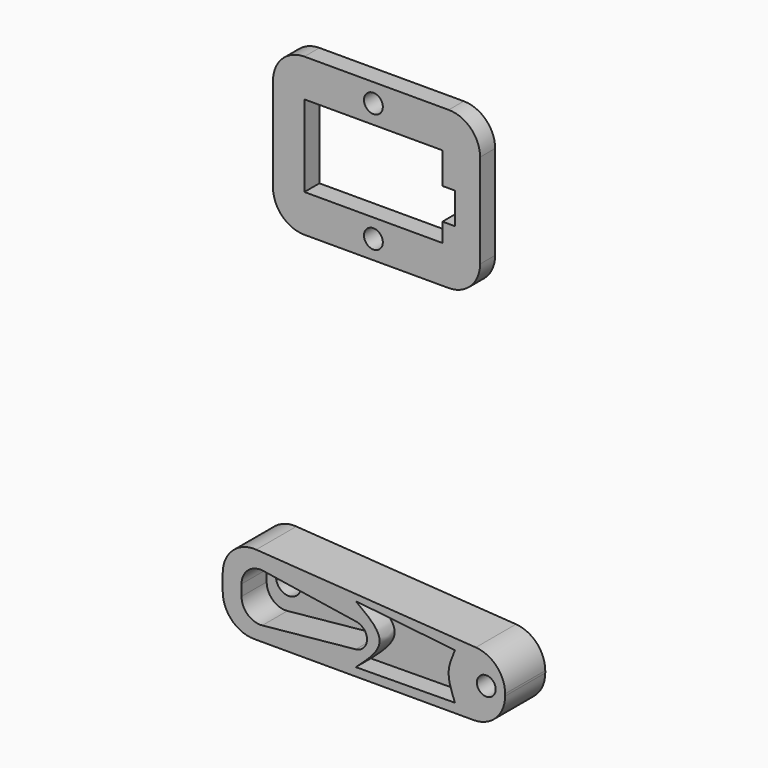
from build123d import *

# Parameters (mm, degrees)
F0_R        = 1.5
F0_R_2      = 2
F1_DEPTH    = 8
F2_R        = 5
F3_R        = 5
F5_DEPTH    = 5
F6_R        = 3
F7_T4_DEPTH = 9.2847060191
F7_T9_DEPTH = 9.5249378106
F9_DEPTH    = 3
F10_W       = 33
F10_H       = 25
F10_R       = 1.5
F11_DEPTH   = 3
F12_R       = 5


# Not quite as in the source:
# - a fillet or chamfer that OpenCascade refuses, or shapes differently, is made with other operations: its cross-section is extruded or revolved along the edge and cut away or added


with BuildPart() as f1:
    # F0 (on Front) → F1 (new body)
    with BuildSketch(Plane.XZ):
        Polygon((-37.012051791, 3), (-37.012051791, -10), (7.987948209, -10), (7.987948209, 0), align=None)
        with Locations((4.987948209, -4.5526479371)):
            Circle(F0_R, mode=Mode.SUBTRACT)
        with Locations((-30.512051791, -3.5)):
            Circle(F0_R_2, mode=Mode.SUBTRACT)
    extrude(amount=F1_DEPTH)

    # F2
    f2_edges = [f1.edges().sort_by_distance(p)[0] for p in [
        (7.987948, -4, 0),
        (7.987948, -4, -10),
    ]]
    fillet(f2_edges, radius=F2_R)

    # F3
    f3_edges = [f1.edges().sort_by_distance(p)[0] for p in [
        (-37.012052, -4, 3),
        (-37.012052, -4, -10),
    ]]
    fillet(f3_edges, radius=F3_R)

    # F4 (on face) → F5 (cut)
    with BuildSketch(Plane.XZ.offset(8)):
        Polygon((-34.012051791, -8), (-14.012051791, -6), (-14.012051791, -2.5333333333), (-34.012051791, 0.5666666667), align=None)
    extrude(amount=-F5_DEPTH, mode=Mode.SUBTRACT)

    # F6
    f6_edges = [f1.edges().sort_by_distance(p)[0] for p in [
        (-34.012052, -5.5, 0.566667),
        (-34.012052, -5.5, -8),
    ]]
    fillet(f6_edges, radius=F6_R)

    # F7: fillet of radius 2 on 2 edges, made by hand


with BuildPart() as f7_tool2:
    # F7_s3 → F7_t4 (new body)
    with BuildSketch(Plane.XZ.offset(8)):
        with BuildLine():
            ThreePointArc((-15.7057098821, -2.2708163292), (-14.493387276, -2.9458095434), (-14.012051791, -4.247215741))
            Line((-14.012051791, -4.247215741), (-14.012051791, -2.5333333333))
            Line((-14.012051791, -2.5333333333), (-15.7057098821, -2.2708163292))
        make_face()
    extrude(amount=-F7_T4_DEPTH)

    split(bisect_by=Plane.XZ, keep=Keep.TOP)


with BuildPart() as f1_1:
    add(f1.part)

    # F7_t1: union F7_tool2
    add(f7_tool2.part)


with BuildPart() as f7_tool7:
    # F7_s8 → F7_t9 (new body)
    with BuildSketch(Plane.XZ.offset(8)):
        with BuildLine():
            ThreePointArc((-15.8130443529, -6.1800992562), (-14.5291467238, -5.5320355173), (-14.012051791, -4.1900248758))
            Line((-14.012051791, -4.1900248758), (-14.012051791, -6))
            Line((-14.012051791, -6), (-15.8130443529, -6.1800992562))
        make_face()
    extrude(amount=-F7_T9_DEPTH)

    split(bisect_by=Plane.XZ, keep=Keep.TOP)


with BuildPart() as f1_2:
    add(f1_1.part)

    # F7_t6: union F7_tool7
    add(f7_tool7.part)

    # F8 (on face) → F9 (cut)
    with BuildSketch(Plane.XZ.offset(8)):
        with BuildLine():
            Line((-0.0122538466, -1.1595856835), (-15.8130443529, 0.5867328375))
            add(Edge.make_bspline(
                [(-15.8130443529, 0.5867328375), (-13.9420993532, -0.7916096765), (-10.1086636088, -3.615737303), (-13.88155084, -6.9601010481), (-15.8130443529, -8.6722160631)],
                knots=[0, 0, 0, 0, 0.4880595696, 1, 1, 1, 1], degree=3))
            Line((-15.8130443529, -8.6722160631), (0, -8.5355339059))
            add(Edge.make_bspline(
                [(-0.0122538466, -1.1595856835), (-0.5061323056, -2.3179393868), (-1.5154357631, -4.6859516385), (-0.5124182093, -7.2339464419), (0, -8.5355339059)],
                knots=[0, 0, 0, 0, 0.4891776198, 1, 1, 1, 1], degree=3))
        make_face()
    extrude(amount=-F9_DEPTH, mode=Mode.SUBTRACT)


with BuildPart() as f11:
    # F10 (on Front) → F11 (new body)
    with BuildSketch(Plane.XZ):
        with Locations((-16.5, 58.4899739623)):
            Rectangle(F10_W, F10_H)
        with Locations((-17, 48.9899739623)):
            Circle(F10_R, mode=Mode.SUBTRACT)
        Polygon((-6, 51.9899739623), (-28, 51.9899739623), (-28, 64.9899739623), (-6, 64.9899739623), (-6, 59.9899739623), (-4, 59.9899739623), (-4, 54.9899739623), (-6, 54.9899739623), align=None, mode=Mode.SUBTRACT)
        with Locations((-17, 67.9899739623)):
            Circle(F10_R, mode=Mode.SUBTRACT)
    extrude(amount=F11_DEPTH)

    # F12
    f12_edges = [f11.edges().sort_by_distance(p)[0] for p in [
        (-33, -1.5, 70.989974),
        (-33, -1.5, 45.989974),
        (0, -1.5, 45.989974),
        (0, -1.5, 70.989974),
    ]]
    fillet(f12_edges, radius=F12_R)


solid = Compound([f1_2.part, f11.part])
